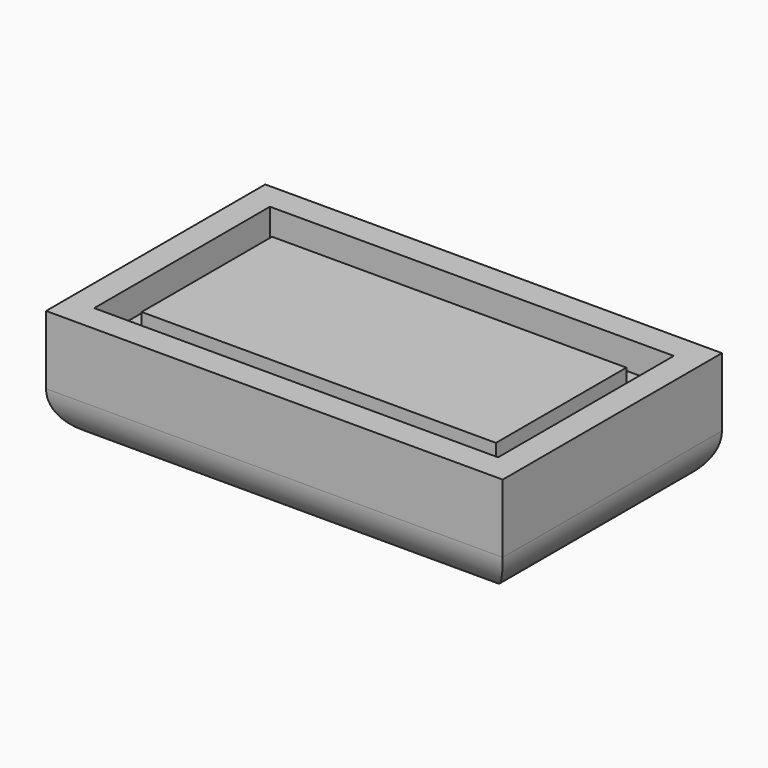
from build123d import *

# Parameters (mm, degrees)
F0_W        = 50.8
F0_H        = 30.48
F0_W_2      = 44.9317246675
F0_H_2      = 24.4365520775
F1_DEPTH    = 6.35
F0_W_3      = 39.4137948751
F0_H_3      = 18.13034527
F2_DEPTH    = 3.175
F3_DEPTH    = 5.588
F4_T1_DEPTH = 76.2
F4_T3_DEPTH = 55.88


# Not quite as in the source:
# - a fillet or chamfer that OpenCascade refuses, or shapes differently, is made with other operations: its cross-section is extruded or revolved along the edge and cut away or added


with BuildPart() as f1:
    # F0 (on Top) → F1 (new body, symmetric)
    with BuildSketch(Plane.XY):
        Rectangle(F0_W, F0_H)
        Rectangle(F0_W_2, F0_H_2, mode=Mode.SUBTRACT)
    extrude(amount=F1_DEPTH, both=True)

    # F0 (on Top) → F2 (join)
    with BuildSketch(Plane.XY):
        Rectangle(F0_W_2, F0_H_2)
        Rectangle(F0_W_3, F0_H_3, mode=Mode.SUBTRACT)
    extrude(amount=F2_DEPTH)

    # F0 (on Top) → F3 (join)
    with BuildSketch(Plane.XY):
        Rectangle(F0_W_3, F0_H_3)
    extrude(amount=F3_DEPTH)

    # F4: fillet of radius 5.08 on 4 edges, made by hand

    # F4_s2 → F4_t1 (cut)
    with BuildSketch(Plane.YZ.offset(-38.1)):
        with BuildLine():
            ThreePointArc((-10.16, -6.35), (-13.7521024484, -4.8621024484), (-15.24, -1.27))
            Line((-15.24, -1.27), (-15.24, -6.35))
            Line((-15.24, -6.35), (-10.16, -6.35))
        make_face()
        with BuildLine():
            ThreePointArc((10.16, -6.35), (13.7521024484, -4.8621024484), (15.24, -1.27))
            Line((15.24, -1.27), (15.24, -6.35))
            Line((15.24, -6.35), (10.16, -6.35))
        make_face()
    extrude(amount=F4_T1_DEPTH, mode=Mode.SUBTRACT)

    # F4_s4 → F4_t3 (cut)
    with BuildSketch(Plane.XZ.offset(-27.94)):
        with BuildLine():
            ThreePointArc((25.4, -1.27), (23.9121024484, -4.8621024484), (20.32, -6.35))
            Line((20.32, -6.35), (25.4, -6.35))
            Line((25.4, -6.35), (25.4, -1.27))
        make_face()
        with BuildLine():
            ThreePointArc((-20.32, -6.35), (-23.9121024484, -4.8621024484), (-25.4, -1.27))
            Line((-25.4, -1.27), (-25.4, -6.35))
            Line((-25.4, -6.35), (-20.32, -6.35))
        make_face()
    extrude(amount=F4_T3_DEPTH, mode=Mode.SUBTRACT)


solid = f1.part
